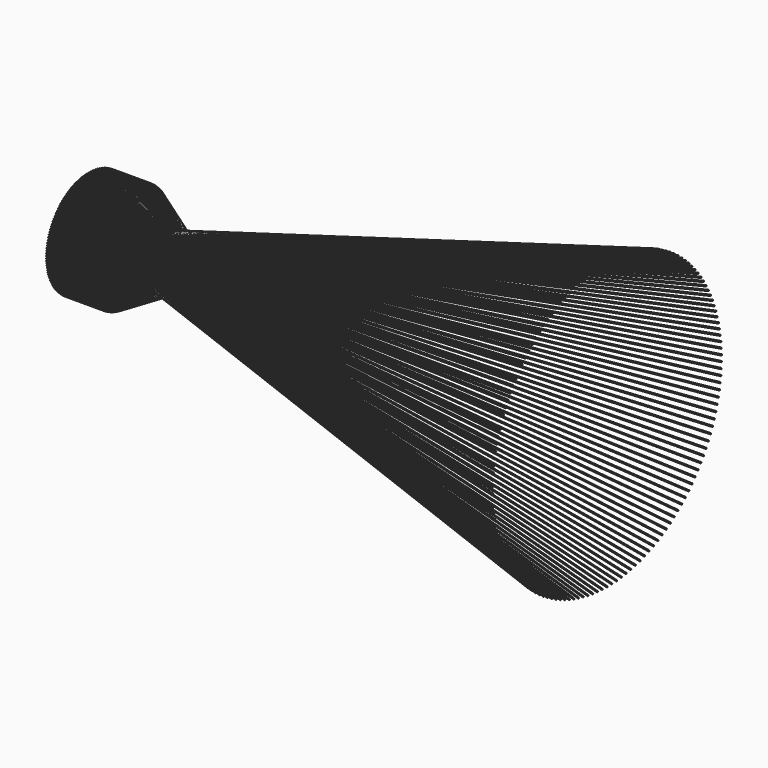
from build123d import *

# Parameters (mm, degrees)
F0_R     = 4.375
F4_COUNT = 150


# Not quite as in the source:
# - the program builds the solid bodies; features that only make, move or delete a surface that nothing else refers to are left out


with BuildPart() as f2:
    # F2: sweep along a path in F1
    with BuildLine(Plane.XZ) as f2_path:
        Line((0, 400.8993184088), (300, 400.8993184088))
        Line((300, 400.8993184088), (647, 200.558775))
        Line((647, 200.558775), (3998.1828001901, 1098.5055))
    # F0 (on Right) → F2 (sweep)
    with BuildSketch(Plane.YZ):
        with Locations((0, 405.492559)):
            Circle(F0_R)
    sweep(path=f2_path.line, transition=Transition.RIGHT)


with BuildPart() as f4_1:
    # F4: instance of F2
    add(f2.part.rotate(Axis((37.2119173408, 0, 0), (1, 0, 0)), 1 * 360 / F4_COUNT))


with BuildPart() as f4_2:
    # F4: instance of F2
    add(f2.part.rotate(Axis((37.2119173408, 0, 0), (1, 0, 0)), 2 * 360 / F4_COUNT))


with BuildPart() as f4_3:
    # F4: instance of F2
    add(f2.part.rotate(Axis((37.2119173408, 0, 0), (1, 0, 0)), 3 * 360 / F4_COUNT))


with BuildPart() as f4_4:
    # F4: instance of F2
    add(f2.part.rotate(Axis((37.2119173408, 0, 0), (1, 0, 0)), 4 * 360 / F4_COUNT))


with BuildPart() as f4_5:
    # F4: instance of F2
    add(f2.part.rotate(Axis((37.2119173408, 0, 0), (1, 0, 0)), 5 * 360 / F4_COUNT))


with BuildPart() as f4_6:
    # F4: instance of F2
    add(f2.part.rotate(Axis((37.2119173408, 0, 0), (1, 0, 0)), 6 * 360 / F4_COUNT))


with BuildPart() as f4_7:
    # F4: instance of F2
    add(f2.part.rotate(Axis((37.2119173408, 0, 0), (1, 0, 0)), 7 * 360 / F4_COUNT))


with BuildPart() as f4_8:
    # F4: instance of F2
    add(f2.part.rotate(Axis((37.2119173408, 0, 0), (1, 0, 0)), 8 * 360 / F4_COUNT))


with BuildPart() as f4_9:
    # F4: instance of F2
    add(f2.part.rotate(Axis((37.2119173408, 0, 0), (1, 0, 0)), 9 * 360 / F4_COUNT))


with BuildPart() as f4_10:
    # F4: instance of F2
    add(f2.part.rotate(Axis((37.2119173408, 0, 0), (1, 0, 0)), 10 * 360 / F4_COUNT))


with BuildPart() as f4_11:
    # F4: instance of F2
    add(f2.part.rotate(Axis((37.2119173408, 0, 0), (1, 0, 0)), 11 * 360 / F4_COUNT))


with BuildPart() as f4_12:
    # F4: instance of F2
    add(f2.part.rotate(Axis((37.2119173408, 0, 0), (1, 0, 0)), 12 * 360 / F4_COUNT))


with BuildPart() as f4_13:
    # F4: instance of F2
    add(f2.part.rotate(Axis((37.2119173408, 0, 0), (1, 0, 0)), 13 * 360 / F4_COUNT))


with BuildPart() as f4_14:
    # F4: instance of F2
    add(f2.part.rotate(Axis((37.2119173408, 0, 0), (1, 0, 0)), 14 * 360 / F4_COUNT))


with BuildPart() as f4_15:
    # F4: instance of F2
    add(f2.part.rotate(Axis((37.2119173408, 0, 0), (1, 0, 0)), 15 * 360 / F4_COUNT))


with BuildPart() as f4_16:
    # F4: instance of F2
    add(f2.part.rotate(Axis((37.2119173408, 0, 0), (1, 0, 0)), 16 * 360 / F4_COUNT))


with BuildPart() as f4_17:
    # F4: instance of F2
    add(f2.part.rotate(Axis((37.2119173408, 0, 0), (1, 0, 0)), 17 * 360 / F4_COUNT))


with BuildPart() as f4_18:
    # F4: instance of F2
    add(f2.part.rotate(Axis((37.2119173408, 0, 0), (1, 0, 0)), 18 * 360 / F4_COUNT))


with BuildPart() as f4_19:
    # F4: instance of F2
    add(f2.part.rotate(Axis((37.2119173408, 0, 0), (1, 0, 0)), 19 * 360 / F4_COUNT))


with BuildPart() as f4_20:
    # F4: instance of F2
    add(f2.part.rotate(Axis((37.2119173408, 0, 0), (1, 0, 0)), 20 * 360 / F4_COUNT))


with BuildPart() as f4_21:
    # F4: instance of F2
    add(f2.part.rotate(Axis((37.2119173408, 0, 0), (1, 0, 0)), 21 * 360 / F4_COUNT))


with BuildPart() as f4_22:
    # F4: instance of F2
    add(f2.part.rotate(Axis((37.2119173408, 0, 0), (1, 0, 0)), 22 * 360 / F4_COUNT))


with BuildPart() as f4_23:
    # F4: instance of F2
    add(f2.part.rotate(Axis((37.2119173408, 0, 0), (1, 0, 0)), 23 * 360 / F4_COUNT))


with BuildPart() as f4_24:
    # F4: instance of F2
    add(f2.part.rotate(Axis((37.2119173408, 0, 0), (1, 0, 0)), 24 * 360 / F4_COUNT))


with BuildPart() as f4_25:
    # F4: instance of F2
    add(f2.part.rotate(Axis((37.2119173408, 0, 0), (1, 0, 0)), 25 * 360 / F4_COUNT))


with BuildPart() as f4_26:
    # F4: instance of F2
    add(f2.part.rotate(Axis((37.2119173408, 0, 0), (1, 0, 0)), 26 * 360 / F4_COUNT))


with BuildPart() as f4_27:
    # F4: instance of F2
    add(f2.part.rotate(Axis((37.2119173408, 0, 0), (1, 0, 0)), 27 * 360 / F4_COUNT))


with BuildPart() as f4_28:
    # F4: instance of F2
    add(f2.part.rotate(Axis((37.2119173408, 0, 0), (1, 0, 0)), 28 * 360 / F4_COUNT))


with BuildPart() as f4_29:
    # F4: instance of F2
    add(f2.part.rotate(Axis((37.2119173408, 0, 0), (1, 0, 0)), 29 * 360 / F4_COUNT))


with BuildPart() as f4_30:
    # F4: instance of F2
    add(f2.part.rotate(Axis((37.2119173408, 0, 0), (1, 0, 0)), 30 * 360 / F4_COUNT))


with BuildPart() as f4_31:
    # F4: instance of F2
    add(f2.part.rotate(Axis((37.2119173408, 0, 0), (1, 0, 0)), 31 * 360 / F4_COUNT))


with BuildPart() as f4_32:
    # F4: instance of F2
    add(f2.part.rotate(Axis((37.2119173408, 0, 0), (1, 0, 0)), 32 * 360 / F4_COUNT))


with BuildPart() as f4_33:
    # F4: instance of F2
    add(f2.part.rotate(Axis((37.2119173408, 0, 0), (1, 0, 0)), 33 * 360 / F4_COUNT))


with BuildPart() as f4_34:
    # F4: instance of F2
    add(f2.part.rotate(Axis((37.2119173408, 0, 0), (1, 0, 0)), 34 * 360 / F4_COUNT))


with BuildPart() as f4_35:
    # F4: instance of F2
    add(f2.part.rotate(Axis((37.2119173408, 0, 0), (1, 0, 0)), 35 * 360 / F4_COUNT))


with BuildPart() as f4_36:
    # F4: instance of F2
    add(f2.part.rotate(Axis((37.2119173408, 0, 0), (1, 0, 0)), 36 * 360 / F4_COUNT))


with BuildPart() as f4_37:
    # F4: instance of F2
    add(f2.part.rotate(Axis((37.2119173408, 0, 0), (1, 0, 0)), 37 * 360 / F4_COUNT))


with BuildPart() as f4_38:
    # F4: instance of F2
    add(f2.part.rotate(Axis((37.2119173408, 0, 0), (1, 0, 0)), 38 * 360 / F4_COUNT))


with BuildPart() as f4_39:
    # F4: instance of F2
    add(f2.part.rotate(Axis((37.2119173408, 0, 0), (1, 0, 0)), 39 * 360 / F4_COUNT))


with BuildPart() as f4_40:
    # F4: instance of F2
    add(f2.part.rotate(Axis((37.2119173408, 0, 0), (1, 0, 0)), 40 * 360 / F4_COUNT))


with BuildPart() as f4_41:
    # F4: instance of F2
    add(f2.part.rotate(Axis((37.2119173408, 0, 0), (1, 0, 0)), 41 * 360 / F4_COUNT))


with BuildPart() as f4_42:
    # F4: instance of F2
    add(f2.part.rotate(Axis((37.2119173408, 0, 0), (1, 0, 0)), 42 * 360 / F4_COUNT))


with BuildPart() as f4_43:
    # F4: instance of F2
    add(f2.part.rotate(Axis((37.2119173408, 0, 0), (1, 0, 0)), 43 * 360 / F4_COUNT))


with BuildPart() as f4_44:
    # F4: instance of F2
    add(f2.part.rotate(Axis((37.2119173408, 0, 0), (1, 0, 0)), 44 * 360 / F4_COUNT))


with BuildPart() as f4_45:
    # F4: instance of F2
    add(f2.part.rotate(Axis((37.2119173408, 0, 0), (1, 0, 0)), 45 * 360 / F4_COUNT))


with BuildPart() as f4_46:
    # F4: instance of F2
    add(f2.part.rotate(Axis((37.2119173408, 0, 0), (1, 0, 0)), 46 * 360 / F4_COUNT))


with BuildPart() as f4_47:
    # F4: instance of F2
    add(f2.part.rotate(Axis((37.2119173408, 0, 0), (1, 0, 0)), 47 * 360 / F4_COUNT))


with BuildPart() as f4_48:
    # F4: instance of F2
    add(f2.part.rotate(Axis((37.2119173408, 0, 0), (1, 0, 0)), 48 * 360 / F4_COUNT))


with BuildPart() as f4_49:
    # F4: instance of F2
    add(f2.part.rotate(Axis((37.2119173408, 0, 0), (1, 0, 0)), 49 * 360 / F4_COUNT))


with BuildPart() as f4_50:
    # F4: instance of F2
    add(f2.part.rotate(Axis((37.2119173408, 0, 0), (1, 0, 0)), 50 * 360 / F4_COUNT))


with BuildPart() as f4_51:
    # F4: instance of F2
    add(f2.part.rotate(Axis((37.2119173408, 0, 0), (1, 0, 0)), 51 * 360 / F4_COUNT))


with BuildPart() as f4_52:
    # F4: instance of F2
    add(f2.part.rotate(Axis((37.2119173408, 0, 0), (1, 0, 0)), 52 * 360 / F4_COUNT))


with BuildPart() as f4_53:
    # F4: instance of F2
    add(f2.part.rotate(Axis((37.2119173408, 0, 0), (1, 0, 0)), 53 * 360 / F4_COUNT))


with BuildPart() as f4_54:
    # F4: instance of F2
    add(f2.part.rotate(Axis((37.2119173408, 0, 0), (1, 0, 0)), 54 * 360 / F4_COUNT))


with BuildPart() as f4_55:
    # F4: instance of F2
    add(f2.part.rotate(Axis((37.2119173408, 0, 0), (1, 0, 0)), 55 * 360 / F4_COUNT))


with BuildPart() as f4_56:
    # F4: instance of F2
    add(f2.part.rotate(Axis((37.2119173408, 0, 0), (1, 0, 0)), 56 * 360 / F4_COUNT))


with BuildPart() as f4_57:
    # F4: instance of F2
    add(f2.part.rotate(Axis((37.2119173408, 0, 0), (1, 0, 0)), 57 * 360 / F4_COUNT))


with BuildPart() as f4_58:
    # F4: instance of F2
    add(f2.part.rotate(Axis((37.2119173408, 0, 0), (1, 0, 0)), 58 * 360 / F4_COUNT))


with BuildPart() as f4_59:
    # F4: instance of F2
    add(f2.part.rotate(Axis((37.2119173408, 0, 0), (1, 0, 0)), 59 * 360 / F4_COUNT))


with BuildPart() as f4_60:
    # F4: instance of F2
    add(f2.part.rotate(Axis((37.2119173408, 0, 0), (1, 0, 0)), 60 * 360 / F4_COUNT))


with BuildPart() as f4_61:
    # F4: instance of F2
    add(f2.part.rotate(Axis((37.2119173408, 0, 0), (1, 0, 0)), 61 * 360 / F4_COUNT))


with BuildPart() as f4_62:
    # F4: instance of F2
    add(f2.part.rotate(Axis((37.2119173408, 0, 0), (1, 0, 0)), 62 * 360 / F4_COUNT))


with BuildPart() as f4_63:
    # F4: instance of F2
    add(f2.part.rotate(Axis((37.2119173408, 0, 0), (1, 0, 0)), 63 * 360 / F4_COUNT))


with BuildPart() as f4_64:
    # F4: instance of F2
    add(f2.part.rotate(Axis((37.2119173408, 0, 0), (1, 0, 0)), 64 * 360 / F4_COUNT))


with BuildPart() as f4_65:
    # F4: instance of F2
    add(f2.part.rotate(Axis((37.2119173408, 0, 0), (1, 0, 0)), 65 * 360 / F4_COUNT))


with BuildPart() as f4_66:
    # F4: instance of F2
    add(f2.part.rotate(Axis((37.2119173408, 0, 0), (1, 0, 0)), 66 * 360 / F4_COUNT))


with BuildPart() as f4_67:
    # F4: instance of F2
    add(f2.part.rotate(Axis((37.2119173408, 0, 0), (1, 0, 0)), 67 * 360 / F4_COUNT))


with BuildPart() as f4_68:
    # F4: instance of F2
    add(f2.part.rotate(Axis((37.2119173408, 0, 0), (1, 0, 0)), 68 * 360 / F4_COUNT))


with BuildPart() as f4_69:
    # F4: instance of F2
    add(f2.part.rotate(Axis((37.2119173408, 0, 0), (1, 0, 0)), 69 * 360 / F4_COUNT))


with BuildPart() as f4_70:
    # F4: instance of F2
    add(f2.part.rotate(Axis((37.2119173408, 0, 0), (1, 0, 0)), 70 * 360 / F4_COUNT))


with BuildPart() as f4_71:
    # F4: instance of F2
    add(f2.part.rotate(Axis((37.2119173408, 0, 0), (1, 0, 0)), 71 * 360 / F4_COUNT))


with BuildPart() as f4_72:
    # F4: instance of F2
    add(f2.part.rotate(Axis((37.2119173408, 0, 0), (1, 0, 0)), 72 * 360 / F4_COUNT))


with BuildPart() as f4_73:
    # F4: instance of F2
    add(f2.part.rotate(Axis((37.2119173408, 0, 0), (1, 0, 0)), 73 * 360 / F4_COUNT))


with BuildPart() as f4_74:
    # F4: instance of F2
    add(f2.part.rotate(Axis((37.2119173408, 0, 0), (1, 0, 0)), 74 * 360 / F4_COUNT))


with BuildPart() as f4_75:
    # F4: instance of F2
    add(f2.part.rotate(Axis((37.2119173408, 0, 0), (1, 0, 0)), 75 * 360 / F4_COUNT))


with BuildPart() as f4_76:
    # F4: instance of F2
    add(f2.part.rotate(Axis((37.2119173408, 0, 0), (1, 0, 0)), 76 * 360 / F4_COUNT))


with BuildPart() as f4_77:
    # F4: instance of F2
    add(f2.part.rotate(Axis((37.2119173408, 0, 0), (1, 0, 0)), 77 * 360 / F4_COUNT))


with BuildPart() as f4_78:
    # F4: instance of F2
    add(f2.part.rotate(Axis((37.2119173408, 0, 0), (1, 0, 0)), 78 * 360 / F4_COUNT))


with BuildPart() as f4_79:
    # F4: instance of F2
    add(f2.part.rotate(Axis((37.2119173408, 0, 0), (1, 0, 0)), 79 * 360 / F4_COUNT))


with BuildPart() as f4_80:
    # F4: instance of F2
    add(f2.part.rotate(Axis((37.2119173408, 0, 0), (1, 0, 0)), 80 * 360 / F4_COUNT))


with BuildPart() as f4_81:
    # F4: instance of F2
    add(f2.part.rotate(Axis((37.2119173408, 0, 0), (1, 0, 0)), 81 * 360 / F4_COUNT))


with BuildPart() as f4_82:
    # F4: instance of F2
    add(f2.part.rotate(Axis((37.2119173408, 0, 0), (1, 0, 0)), 82 * 360 / F4_COUNT))


with BuildPart() as f4_83:
    # F4: instance of F2
    add(f2.part.rotate(Axis((37.2119173408, 0, 0), (1, 0, 0)), 83 * 360 / F4_COUNT))


with BuildPart() as f4_84:
    # F4: instance of F2
    add(f2.part.rotate(Axis((37.2119173408, 0, 0), (1, 0, 0)), 84 * 360 / F4_COUNT))


with BuildPart() as f4_85:
    # F4: instance of F2
    add(f2.part.rotate(Axis((37.2119173408, 0, 0), (1, 0, 0)), 85 * 360 / F4_COUNT))


with BuildPart() as f4_86:
    # F4: instance of F2
    add(f2.part.rotate(Axis((37.2119173408, 0, 0), (1, 0, 0)), 86 * 360 / F4_COUNT))


with BuildPart() as f4_87:
    # F4: instance of F2
    add(f2.part.rotate(Axis((37.2119173408, 0, 0), (1, 0, 0)), 87 * 360 / F4_COUNT))


with BuildPart() as f4_88:
    # F4: instance of F2
    add(f2.part.rotate(Axis((37.2119173408, 0, 0), (1, 0, 0)), 88 * 360 / F4_COUNT))


with BuildPart() as f4_89:
    # F4: instance of F2
    add(f2.part.rotate(Axis((37.2119173408, 0, 0), (1, 0, 0)), 89 * 360 / F4_COUNT))


with BuildPart() as f4_90:
    # F4: instance of F2
    add(f2.part.rotate(Axis((37.2119173408, 0, 0), (1, 0, 0)), 90 * 360 / F4_COUNT))


with BuildPart() as f4_91:
    # F4: instance of F2
    add(f2.part.rotate(Axis((37.2119173408, 0, 0), (1, 0, 0)), 91 * 360 / F4_COUNT))


with BuildPart() as f4_92:
    # F4: instance of F2
    add(f2.part.rotate(Axis((37.2119173408, 0, 0), (1, 0, 0)), 92 * 360 / F4_COUNT))


with BuildPart() as f4_93:
    # F4: instance of F2
    add(f2.part.rotate(Axis((37.2119173408, 0, 0), (1, 0, 0)), 93 * 360 / F4_COUNT))


with BuildPart() as f4_94:
    # F4: instance of F2
    add(f2.part.rotate(Axis((37.2119173408, 0, 0), (1, 0, 0)), 94 * 360 / F4_COUNT))


with BuildPart() as f4_95:
    # F4: instance of F2
    add(f2.part.rotate(Axis((37.2119173408, 0, 0), (1, 0, 0)), 95 * 360 / F4_COUNT))


with BuildPart() as f4_96:
    # F4: instance of F2
    add(f2.part.rotate(Axis((37.2119173408, 0, 0), (1, 0, 0)), 96 * 360 / F4_COUNT))


with BuildPart() as f4_97:
    # F4: instance of F2
    add(f2.part.rotate(Axis((37.2119173408, 0, 0), (1, 0, 0)), 97 * 360 / F4_COUNT))


with BuildPart() as f4_98:
    # F4: instance of F2
    add(f2.part.rotate(Axis((37.2119173408, 0, 0), (1, 0, 0)), 98 * 360 / F4_COUNT))


with BuildPart() as f4_99:
    # F4: instance of F2
    add(f2.part.rotate(Axis((37.2119173408, 0, 0), (1, 0, 0)), 99 * 360 / F4_COUNT))


with BuildPart() as f4_100:
    # F4: instance of F2
    add(f2.part.rotate(Axis((37.2119173408, 0, 0), (1, 0, 0)), 100 * 360 / F4_COUNT))


with BuildPart() as f4_101:
    # F4: instance of F2
    add(f2.part.rotate(Axis((37.2119173408, 0, 0), (1, 0, 0)), 101 * 360 / F4_COUNT))


with BuildPart() as f4_102:
    # F4: instance of F2
    add(f2.part.rotate(Axis((37.2119173408, 0, 0), (1, 0, 0)), 102 * 360 / F4_COUNT))


with BuildPart() as f4_103:
    # F4: instance of F2
    add(f2.part.rotate(Axis((37.2119173408, 0, 0), (1, 0, 0)), 103 * 360 / F4_COUNT))


with BuildPart() as f4_104:
    # F4: instance of F2
    add(f2.part.rotate(Axis((37.2119173408, 0, 0), (1, 0, 0)), 104 * 360 / F4_COUNT))


with BuildPart() as f4_105:
    # F4: instance of F2
    add(f2.part.rotate(Axis((37.2119173408, 0, 0), (1, 0, 0)), 105 * 360 / F4_COUNT))


with BuildPart() as f4_106:
    # F4: instance of F2
    add(f2.part.rotate(Axis((37.2119173408, 0, 0), (1, 0, 0)), 106 * 360 / F4_COUNT))


with BuildPart() as f4_107:
    # F4: instance of F2
    add(f2.part.rotate(Axis((37.2119173408, 0, 0), (1, 0, 0)), 107 * 360 / F4_COUNT))


with BuildPart() as f4_108:
    # F4: instance of F2
    add(f2.part.rotate(Axis((37.2119173408, 0, 0), (1, 0, 0)), 108 * 360 / F4_COUNT))


with BuildPart() as f4_109:
    # F4: instance of F2
    add(f2.part.rotate(Axis((37.2119173408, 0, 0), (1, 0, 0)), 109 * 360 / F4_COUNT))


with BuildPart() as f4_110:
    # F4: instance of F2
    add(f2.part.rotate(Axis((37.2119173408, 0, 0), (1, 0, 0)), 110 * 360 / F4_COUNT))


with BuildPart() as f4_111:
    # F4: instance of F2
    add(f2.part.rotate(Axis((37.2119173408, 0, 0), (1, 0, 0)), 111 * 360 / F4_COUNT))


with BuildPart() as f4_112:
    # F4: instance of F2
    add(f2.part.rotate(Axis((37.2119173408, 0, 0), (1, 0, 0)), 112 * 360 / F4_COUNT))


with BuildPart() as f4_113:
    # F4: instance of F2
    add(f2.part.rotate(Axis((37.2119173408, 0, 0), (1, 0, 0)), 113 * 360 / F4_COUNT))


with BuildPart() as f4_114:
    # F4: instance of F2
    add(f2.part.rotate(Axis((37.2119173408, 0, 0), (1, 0, 0)), 114 * 360 / F4_COUNT))


with BuildPart() as f4_115:
    # F4: instance of F2
    add(f2.part.rotate(Axis((37.2119173408, 0, 0), (1, 0, 0)), 115 * 360 / F4_COUNT))


with BuildPart() as f4_116:
    # F4: instance of F2
    add(f2.part.rotate(Axis((37.2119173408, 0, 0), (1, 0, 0)), 116 * 360 / F4_COUNT))


with BuildPart() as f4_117:
    # F4: instance of F2
    add(f2.part.rotate(Axis((37.2119173408, 0, 0), (1, 0, 0)), 117 * 360 / F4_COUNT))


with BuildPart() as f4_118:
    # F4: instance of F2
    add(f2.part.rotate(Axis((37.2119173408, 0, 0), (1, 0, 0)), 118 * 360 / F4_COUNT))


with BuildPart() as f4_119:
    # F4: instance of F2
    add(f2.part.rotate(Axis((37.2119173408, 0, 0), (1, 0, 0)), 119 * 360 / F4_COUNT))


with BuildPart() as f4_120:
    # F4: instance of F2
    add(f2.part.rotate(Axis((37.2119173408, 0, 0), (1, 0, 0)), 120 * 360 / F4_COUNT))


with BuildPart() as f4_121:
    # F4: instance of F2
    add(f2.part.rotate(Axis((37.2119173408, 0, 0), (1, 0, 0)), 121 * 360 / F4_COUNT))


with BuildPart() as f4_122:
    # F4: instance of F2
    add(f2.part.rotate(Axis((37.2119173408, 0, 0), (1, 0, 0)), 122 * 360 / F4_COUNT))


with BuildPart() as f4_123:
    # F4: instance of F2
    add(f2.part.rotate(Axis((37.2119173408, 0, 0), (1, 0, 0)), 123 * 360 / F4_COUNT))


with BuildPart() as f4_124:
    # F4: instance of F2
    add(f2.part.rotate(Axis((37.2119173408, 0, 0), (1, 0, 0)), 124 * 360 / F4_COUNT))


with BuildPart() as f4_125:
    # F4: instance of F2
    add(f2.part.rotate(Axis((37.2119173408, 0, 0), (1, 0, 0)), 125 * 360 / F4_COUNT))


with BuildPart() as f4_126:
    # F4: instance of F2
    add(f2.part.rotate(Axis((37.2119173408, 0, 0), (1, 0, 0)), 126 * 360 / F4_COUNT))


with BuildPart() as f4_127:
    # F4: instance of F2
    add(f2.part.rotate(Axis((37.2119173408, 0, 0), (1, 0, 0)), 127 * 360 / F4_COUNT))


with BuildPart() as f4_128:
    # F4: instance of F2
    add(f2.part.rotate(Axis((37.2119173408, 0, 0), (1, 0, 0)), 128 * 360 / F4_COUNT))


with BuildPart() as f4_129:
    # F4: instance of F2
    add(f2.part.rotate(Axis((37.2119173408, 0, 0), (1, 0, 0)), 129 * 360 / F4_COUNT))


with BuildPart() as f4_130:
    # F4: instance of F2
    add(f2.part.rotate(Axis((37.2119173408, 0, 0), (1, 0, 0)), 130 * 360 / F4_COUNT))


with BuildPart() as f4_131:
    # F4: instance of F2
    add(f2.part.rotate(Axis((37.2119173408, 0, 0), (1, 0, 0)), 131 * 360 / F4_COUNT))


with BuildPart() as f4_132:
    # F4: instance of F2
    add(f2.part.rotate(Axis((37.2119173408, 0, 0), (1, 0, 0)), 132 * 360 / F4_COUNT))


with BuildPart() as f4_133:
    # F4: instance of F2
    add(f2.part.rotate(Axis((37.2119173408, 0, 0), (1, 0, 0)), 133 * 360 / F4_COUNT))


with BuildPart() as f4_134:
    # F4: instance of F2
    add(f2.part.rotate(Axis((37.2119173408, 0, 0), (1, 0, 0)), 134 * 360 / F4_COUNT))


with BuildPart() as f4_135:
    # F4: instance of F2
    add(f2.part.rotate(Axis((37.2119173408, 0, 0), (1, 0, 0)), 135 * 360 / F4_COUNT))


with BuildPart() as f4_136:
    # F4: instance of F2
    add(f2.part.rotate(Axis((37.2119173408, 0, 0), (1, 0, 0)), 136 * 360 / F4_COUNT))


with BuildPart() as f4_137:
    # F4: instance of F2
    add(f2.part.rotate(Axis((37.2119173408, 0, 0), (1, 0, 0)), 137 * 360 / F4_COUNT))


with BuildPart() as f4_138:
    # F4: instance of F2
    add(f2.part.rotate(Axis((37.2119173408, 0, 0), (1, 0, 0)), 138 * 360 / F4_COUNT))


with BuildPart() as f4_139:
    # F4: instance of F2
    add(f2.part.rotate(Axis((37.2119173408, 0, 0), (1, 0, 0)), 139 * 360 / F4_COUNT))


with BuildPart() as f4_140:
    # F4: instance of F2
    add(f2.part.rotate(Axis((37.2119173408, 0, 0), (1, 0, 0)), 140 * 360 / F4_COUNT))


with BuildPart() as f4_141:
    # F4: instance of F2
    add(f2.part.rotate(Axis((37.2119173408, 0, 0), (1, 0, 0)), 141 * 360 / F4_COUNT))


with BuildPart() as f4_142:
    # F4: instance of F2
    add(f2.part.rotate(Axis((37.2119173408, 0, 0), (1, 0, 0)), 142 * 360 / F4_COUNT))


with BuildPart() as f4_143:
    # F4: instance of F2
    add(f2.part.rotate(Axis((37.2119173408, 0, 0), (1, 0, 0)), 143 * 360 / F4_COUNT))


with BuildPart() as f4_144:
    # F4: instance of F2
    add(f2.part.rotate(Axis((37.2119173408, 0, 0), (1, 0, 0)), 144 * 360 / F4_COUNT))


with BuildPart() as f4_145:
    # F4: instance of F2
    add(f2.part.rotate(Axis((37.2119173408, 0, 0), (1, 0, 0)), 145 * 360 / F4_COUNT))


with BuildPart() as f4_146:
    # F4: instance of F2
    add(f2.part.rotate(Axis((37.2119173408, 0, 0), (1, 0, 0)), 146 * 360 / F4_COUNT))


with BuildPart() as f4_147:
    # F4: instance of F2
    add(f2.part.rotate(Axis((37.2119173408, 0, 0), (1, 0, 0)), 147 * 360 / F4_COUNT))


with BuildPart() as f4_148:
    # F4: instance of F2
    add(f2.part.rotate(Axis((37.2119173408, 0, 0), (1, 0, 0)), 148 * 360 / F4_COUNT))


with BuildPart() as f4_149:
    # F4: instance of F2
    add(f2.part.rotate(Axis((37.2119173408, 0, 0), (1, 0, 0)), 149 * 360 / F4_COUNT))


solid = Compound([f2.part, f4_1.part, f4_2.part, f4_3.part, f4_4.part, f4_5.part, f4_6.part, f4_7.part, f4_8.part, f4_9.part, f4_10.part, f4_11.part, f4_12.part, f4_13.part, f4_14.part, f4_15.part, f4_16.part, f4_17.part, f4_18.part, f4_19.part, f4_20.part, f4_21.part, f4_22.part, f4_23.part, f4_24.part, f4_25.part, f4_26.part, f4_27.part, f4_28.part, f4_29.part, f4_30.part, f4_31.part, f4_32.part, f4_33.part, f4_34.part, f4_35.part, f4_36.part, f4_37.part, f4_38.part, f4_39.part, f4_40.part, f4_41.part, f4_42.part, f4_43.part, f4_44.part, f4_45.part, f4_46.part, f4_47.part, f4_48.part, f4_49.part, f4_50.part, f4_51.part, f4_52.part, f4_53.part, f4_54.part, f4_55.part, f4_56.part, f4_57.part, f4_58.part, f4_59.part, f4_60.part, f4_61.part, f4_62.part, f4_63.part, f4_64.part, f4_65.part, f4_66.part, f4_67.part, f4_68.part, f4_69.part, f4_70.part, f4_71.part, f4_72.part, f4_73.part, f4_74.part, f4_75.part, f4_76.part, f4_77.part, f4_78.part, f4_79.part, f4_80.part, f4_81.part, f4_82.part, f4_83.part, f4_84.part, f4_85.part, f4_86.part, f4_87.part, f4_88.part, f4_89.part, f4_90.part, f4_91.part, f4_92.part, f4_93.part, f4_94.part, f4_95.part, f4_96.part, f4_97.part, f4_98.part, f4_99.part, f4_100.part, f4_101.part, f4_102.part, f4_103.part, f4_104.part, f4_105.part, f4_106.part, f4_107.part, f4_108.part, f4_109.part, f4_110.part, f4_111.part, f4_112.part, f4_113.part, f4_114.part, f4_115.part, f4_116.part, f4_117.part, f4_118.part, f4_119.part, f4_120.part, f4_121.part, f4_122.part, f4_123.part, f4_124.part, f4_125.part, f4_126.part, f4_127.part, f4_128.part, f4_129.part, f4_130.part, f4_131.part, f4_132.part, f4_133.part, f4_134.part, f4_135.part, f4_136.part, f4_137.part, f4_138.part, f4_139.part, f4_140.part, f4_141.part, f4_142.part, f4_143.part, f4_144.part, f4_145.part, f4_146.part, f4_147.part, f4_148.part, f4_149.part])
